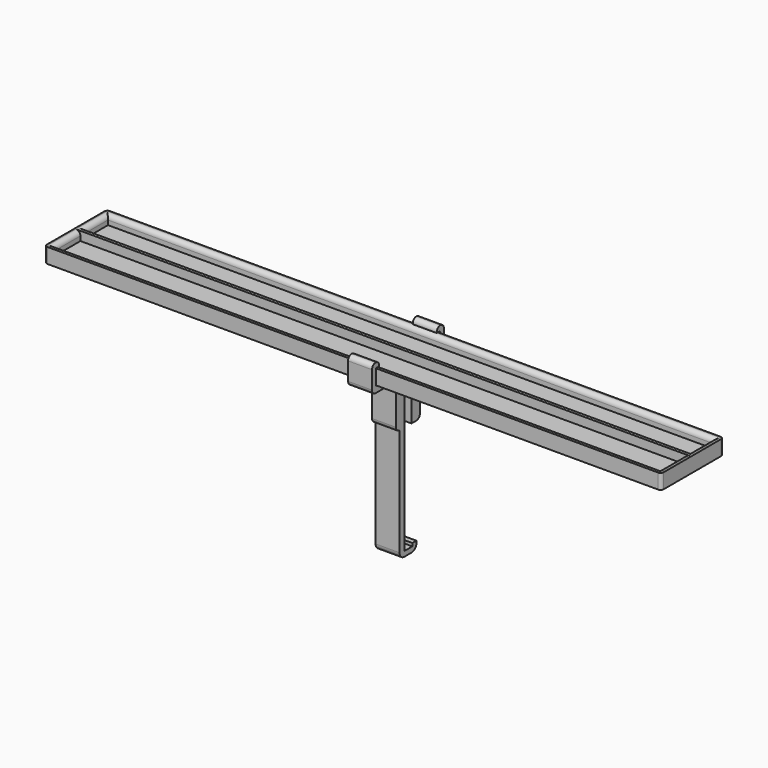
from build123d import *

# Parameters (mm, degrees)
F0_W      = 206
F0_H      = 26
F1_DEPTH  = 2
F2_W      = 206
F2_H      = 26
F2_W_2    = 202
F2_H_2    = 10.5
F3_DEPTH  = 3
F4_R      = 1.5
F5_R      = 1
F7_DEPTH  = 8
F8_W      = 8
F8_H      = 3.525
F9_DEPTH  = 15
F10_R     = 1.49999
F11_W     = 8
F11_H     = 2.025
F12_DEPTH = 38
F13_W     = 8
F13_H     = 1.7
F14_DEPTH = 5
F15_W     = 8
F15_H     = 1.7
F16_DEPTH = 1
F17_R     = 2


# Not quite as in the source:
# - a fillet or chamfer is up to 0.001 mm smaller than in the source, because OpenCascade refuses the exact size


with BuildPart() as f1:
    # F0 (on Top) → F1 (new body)
    with BuildSketch(Plane.XY):
        Rectangle(F0_W, F0_H)
    extrude(amount=F1_DEPTH)

    # F2 (on face) → F3 (join)
    with BuildSketch(Plane.XY.offset(2)):
        Rectangle(F2_W, F2_H)
        with Locations((0, -5.75)):
            Rectangle(F2_W_2, F2_H_2, mode=Mode.SUBTRACT)
        with Locations((0, 5.75)):
            Rectangle(F2_W_2, F2_H_2, mode=Mode.SUBTRACT)
    extrude(amount=F3_DEPTH)

    # F4
    f4_edges = [f1.edges().sort_by_distance(p)[0] for p in [
        (-101, 5.75, 5),
        (0, 11, 5),
        (-101, -5.75, 5),
        (0, -11, 5),
        (101, 5.75, 5),
        (101, -5.75, 5),
    ]]
    fillet(f4_edges, radius=F4_R)

    # F5
    f5_edges = [f1.edges().sort_by_distance(p)[0] for p in [
        (103, 13, 2.5),
        (103, -13, 2.5),
        (-103, -13, 2.5),
        (-103, 13, 2.5),
    ]]
    fillet(f5_edges, radius=F5_R)


with BuildPart() as f7:
    # F6 (on Right) → F7 (new body)
    with BuildSketch(Plane.YZ):
        Polygon((13, 0), (12, 0), (-12, 0), (-13, 0), (-13.3, 0), (-13.3, 5.3), (-12, 5.3), (-12, 7), (-15, 7), (-15, -2), (-12, -2), (12, -2), (15, -2), (15, 7), (12, 7), (12, 5.3), (13.3, 5.3), (13.3, 0), align=None)
    extrude(amount=F7_DEPTH)

    # F8 (on face) → F9 (join)
    with BuildSketch(Plane(origin=(0, 0, -2), x_dir=(1, 0, 0), z_dir=(0, 0, -1))):
        with Locations((4, 3.2375)):
            Rectangle(F8_W, F8_H)
        with Locations((4, -3.2375)):
            Rectangle(F8_W, F8_H)
    extrude(amount=F9_DEPTH)

    # F10 (radius 1.5 in the source; OpenCascade refuses exactly that, so slightly less here)
    f10_edges = [f7.edges().sort_by_distance(p)[0] for p in [
        (4, -15, 7),
        (4, -15, -2),
        (4, 15, 7),
        (4, 15, -2),
        (4, 5, -2),
        (4, -5, -2),
        (4, -5, -17),
        (4, 5, -17),
        (4, -12, 7),
        (4, 12, 7),
    ]]
    fillet(f10_edges, radius=F10_R)

    # F11 (on face) → F12 (join)
    with BuildSketch(Plane(origin=(0, 0, -17), x_dir=(1, 0, 0), z_dir=(0, 0, -1))):
        with Locations((4, 2.4875)):
            Rectangle(F11_W, F11_H)
    extrude(amount=F12_DEPTH)

    # F13 (on face) → F14 (join)
    with BuildSketch(Plane(origin=(0, -1.475, 0), x_dir=(-1, 0, 0), z_dir=(0, 1, 0))):
        with Locations((-4, -54.15)):
            Rectangle(F13_W, F13_H)
    extrude(amount=F14_DEPTH)

    # F15 (on face) → F16 (join)
    with BuildSketch(Plane.XY.offset(-53.3)):
        with Locations((4, 2.675)):
            Rectangle(F15_W, F15_H)
    extrude(amount=F16_DEPTH)

    # F17
    f17_edges = [f7.edges().sort_by_distance(p)[0] for p in [
        (4, 3.525, -55),
        (4, -3.5, -55),
    ]]
    fillet(f17_edges, radius=F17_R)


solid = Compound([f1.part, f7.part])
